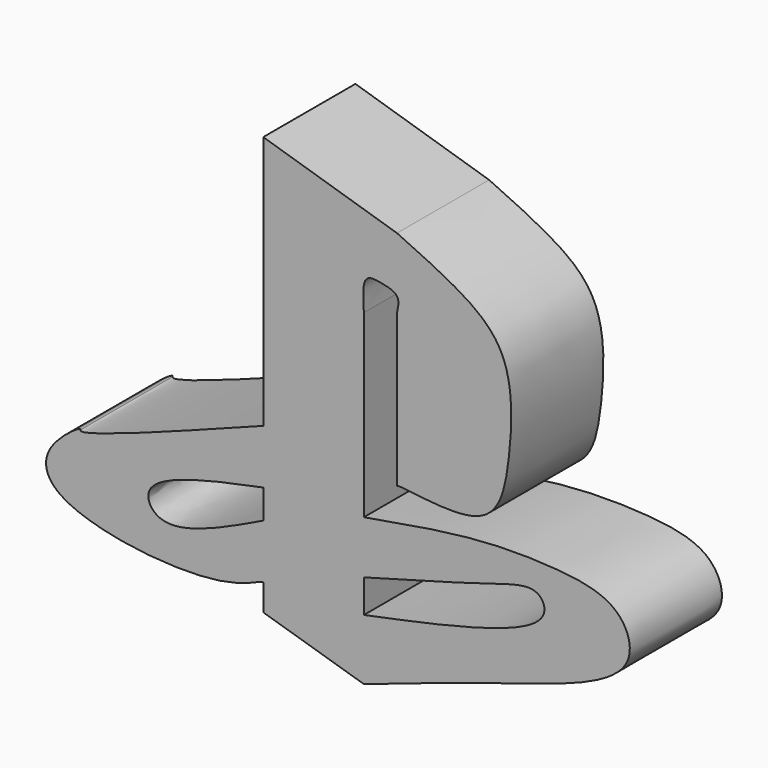
from build123d import *

# Parameters (mm, degrees)
F1_DEPTH = 25.4


with BuildPart() as f1:
    # F0 (on Front) → F1 (new body)
    with BuildSketch(Plane.XZ):
        with BuildLine():
            Line((-15.3303835541, -41.0270281136), (-15.3303835541, -46.5751625597))
            Line((-15.3303835541, -46.5751625597), (6.8621719256, -53.2913357019))
            Line((6.8621719256, -53.2913357019), (6.8621719256, -39.8589968681))
            Line((6.8621719256, -39.8589968681), (6.8621719256, -32.5588136911))
            Line((6.8621719256, -32.5588136911), (6.8621719256, -20.8785217255))
            Line((6.8621719256, -20.8785217255), (6.8621719256, 18.8344717026))
            add(Edge.make_bspline(
                [(14.1623523086, 21.1705304682), (14.4264375928, 22.3843703264), (14.9776139766, 24.917793821), (10.6853785059, 25.8987456687), (6.3392125116, 26.5024260876), (6.6678848939, 21.683228331), (6.8621719256, 18.8344717026)],
                knots=[0, 0, 0, 0, 0.220366293, 0.4599298172, 0.6807500769, 1, 1, 1, 1], degree=3))
            Line((14.1623523086, 21.1705304682), (14.1623523086, -12.4103110284))
            add(Edge.make_bspline(
                [(14.1623523086, 36.6469174623), (18.1059212038, 34.8455598925), (26.2188057649, 31.1397273318), (40.2392334697, 22.2058630586), (39.3449689326, 0.2448984557), (35.4080251913, -16.7285134667), (15.009821869, -11.9220096004), (14.1623523086, -12.4103110284)],
                knots=[0, 0, 0, 0, 0.1771529227, 0.3644468373, 0.5865030589, 0.7722885895, 0.9737711488, 0.9737711488, 0.9737711488, 0.9737711488], degree=3))
            Line((14.1623523086, 36.6469174623), (-15.3303835541, 45.7038161606))
            Line((-15.3303835541, 45.7038161606), (-15.3303835541, -10.3662600741))
            Line((-15.3303835541, -10.3662600741), (-15.3303835541, -22.3385579884))
            Line((-15.3303835541, -22.3385579884), (-15.3303835541, -28.7627186626))
            Line((-15.3303835541, -28.7627186626), (-15.3303835541, -40.7350212336))
            add(Edge.make_bspline(
                [(-15.3303835541, -40.7350212336), (-15.2712927491, -40.7837414321), (-15.3008381516, -40.9053847728), (-15.3303835541, -41.0270281136)],
                knots=[0.9760015175, 0.9760015175, 0.9760015175, 0.9760015175, 1, 1, 1, 1], degree=3))
        make_face()
        with BuildLine():
            Line((-15.3303835541, -40.7350212336), (-15.3303835541, -41.0270281136))
            add(Edge.make_bspline(
                [(-15.3303835541, -40.7350212336), (-15.2712927491, -40.7837414321), (-15.3008381516, -40.9053847728), (-15.3303835541, -41.0270281136)],
                knots=[0.9760015175, 0.9760015175, 0.9760015175, 0.9760015175, 1, 1, 1, 1], degree=3))
        make_face()
        with BuildLine():
            Line((6.8621719256, -39.8589968681), (6.8621719256, -53.2913357019))
            add(Edge.make_bspline(
                [(6.8621719256, -20.8785217255), (15.3042216434, -19.378819076), (31.0173786315, -16.5874278907), (49.0894784823, -16.7967105962), (63.6993881596, -18.9897924504), (68.6223083484, -33.9934598901), (36.3748012962, -43.1794652259), (16.9488069817, -49.8353661932), (6.8621719256, -53.2913357019)],
                knots=[0, 0, 0, 0, 0.1832299895, 0.3410453251, 0.4759333054, 0.5897297817, 0.7869737889, 1, 1, 1, 1], degree=3))
            Line((6.8621719256, -20.8785217255), (6.8621719256, -32.5588136911))
            add(Edge.make_bspline(
                [(6.8621719256, -32.5588136911), (17.075486717, -29.783960217), (33.370052461, -25.3568928752), (45.3413435566, -21.2588853056), (49.396785617, -31.105994635), (25.1915382166, -36.0870810059), (6.8621719256, -39.8589968681)],
                knots=[0, 0, 0, 0, 0.3155094949, 0.5033713649, 0.6239291418, 1, 1, 1, 1], degree=3))
        make_face()
        with BuildLine():
            add(Edge.make_bspline(
                [(-15.3303835541, -10.3662600741), (-35.2206782898, -17.9375768513), (-56.7564818958, -26.1352628746), (-55.0956742109, -23.3134101991), (-64.396064605, -29.5675464926), (-62.7832606242, -42.0369715173), (-24.8258652624, -46.3806221426), (-15.6559974585, -40.4665535073), (-15.3303835541, -40.7350212336)],
                knots=[0, 0, 0, 0, 0.2900837403, 0.3140821462, 0.443471427, 0.5740686868, 0.843760307, 0.9760015175, 0.9760015175, 0.9760015175, 0.9760015175], degree=3))
            Line((-15.3303835541, -40.7350212336), (-15.3303835541, -28.7627186626))
            add(Edge.make_bspline(
                [(-15.3303835541, -22.3385579884), (-27.010916279, -24.7241738586), (-43.9353309171, -28.1807929276), (-37.4681885021, -39.4346237824), (-24.267423007, -33.070970421), (-15.3303835541, -28.7627186626)],
                knots=[0, 0, 0, 0, 0.4184182917, 0.6062638433, 1, 1, 1, 1], degree=3))
            Line((-15.3303835541, -22.3385579884), (-15.3303835541, -10.3662600741))
        make_face()
    extrude(amount=F1_DEPTH)


solid = f1.part
